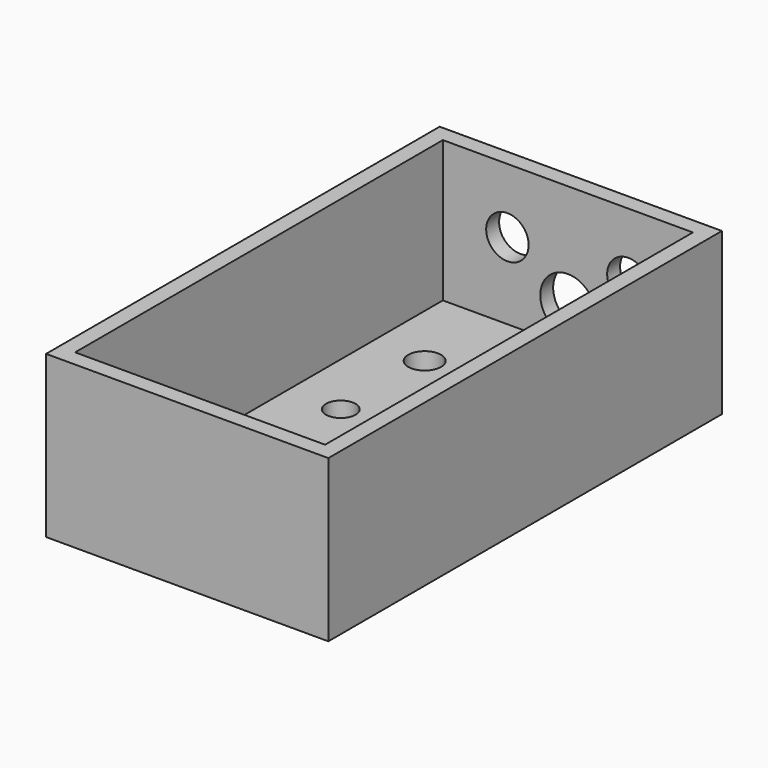
from build123d import *

# Parameters (mm, degrees)
F0_W         = 70
F0_H         = 122
F1_DEPTH     = 40
F2_W         = 62
F2_H         = 114
F3_DEPTH     = 35
F4_R         = 4.071875
F4_R_2       = 3.675
F4_R_3       = 6.35
F5_DEPTH     = 25
F6_R         = 6.85
F6_R_2       = 5.2625
F7_DEPTH     = 25
F9_TEXT_SIZE = 6.9444444444
F10_DEPTH    = 2


# Not quite as in the source:
# - Text() gives the source's letters only with a copy of the font that has no kerning and outlines rounded to 1/6400 em; it was checked with that copy


with BuildPart() as f1:
    # F0 (on Top) → F1 (new body)
    with BuildSketch(Plane.XY):
        Rectangle(F0_W, F0_H)
    extrude(amount=F1_DEPTH)

    # F2 (on face) → F3 (cut)
    with BuildSketch(Plane.XY.offset(40)):
        Rectangle(F2_W, F2_H)
    extrude(amount=-F3_DEPTH, mode=Mode.SUBTRACT)

    # F4 (on face) → F5 (cut)
    with BuildSketch(Plane.XY.offset(5)):
        with Locations((-17.9119046929, 35)):
            Circle(F4_R)
        with Locations((0, 35)):
            Circle(F4_R)
        with Locations((17.9119046929, 35)):
            Circle(F4_R)
        with Locations((17.9119046929, 9)):
            Circle(F4_R_2)
        with Locations((0, -38)):
            Circle(F4_R_3)
        with Locations((-17.9119046929, 9)):
            Circle(F4_R_2)
    extrude(amount=-F5_DEPTH, mode=Mode.SUBTRACT)

    # F6 (on face) → F7 (cut)
    with BuildSketch(Plane.XZ.offset(-57)):
        with Locations((0, 14)):
            Circle(F6_R)
        with Locations((15, 24)):
            Circle(F6_R_2)
        with Locations((-15, 24)):
            Circle(F6_R_2)
    extrude(amount=-F7_DEPTH, mode=Mode.SUBTRACT)

    # F9 (on face) → F10 (cut)
    with BuildSketch(Plane(origin=(0, 0, 0), x_dir=(1, 0, 0), z_dir=(0, 0, -1))):
        with Locations(Location((29.3945663914, -20), (0, 0, 180))):
            Text('VOL', F9_TEXT_SIZE, font='Open Sans', font_style=FontStyle.BOLD, text_align=(TextAlign.LEFT, TextAlign.BOTTOM))
        with Locations(Location((9.5616319444, -20), (0, 0, 180))):
            Text('TONE', F9_TEXT_SIZE, font='Open Sans', font_style=FontStyle.BOLD, text_align=(TextAlign.LEFT, TextAlign.BOTTOM))
        with Locations(Location((-11.8034205581, -20), (0, 0, 180))):
            Text('GAIN', F9_TEXT_SIZE, font='Open Sans', font_style=FontStyle.BOLD, text_align=(TextAlign.LEFT, TextAlign.BOTTOM))
    extrude(amount=-F10_DEPTH, mode=Mode.SUBTRACT)


solid = f1.part
